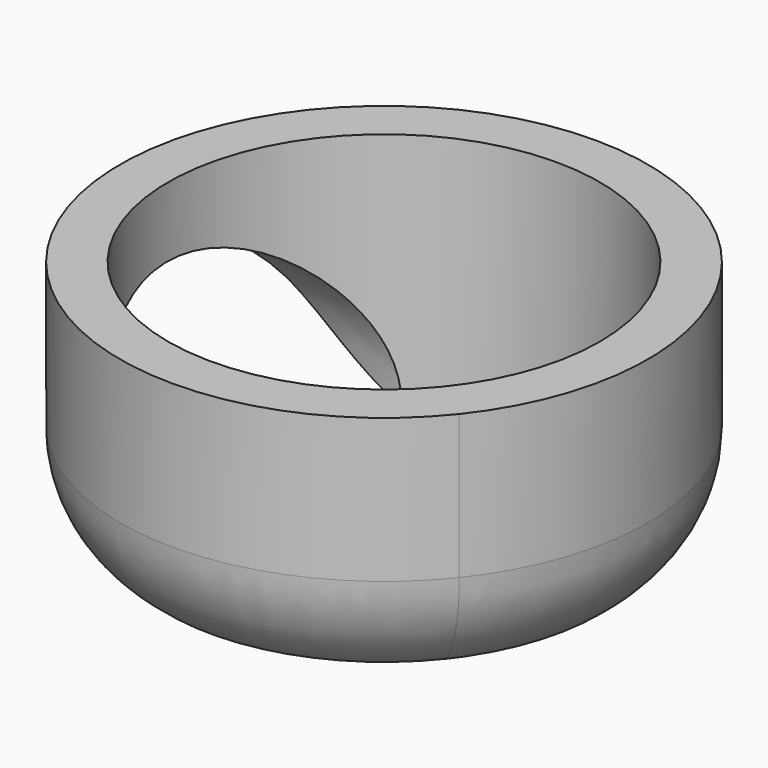
from build123d import *

# Parameters (mm, degrees)
F1_DEPTH    = 10
F3_DEPTH    = 25
F4_DEPTH    = 25
F5_T2_ANGLE = 228.5604314435
F5_T4_ANGLE = 149.7338838055


# Not quite as in the source:
# - a fillet or chamfer that OpenCascade refuses, or shapes differently, is made with other operations: its cross-section is extruded or revolved along the edge and cut away or added


with BuildPart() as f1:
    # F0 (on Top) → F1 (new body)
    with BuildSketch(Plane.XY):
        with BuildLine():
            ThreePointArc((7.4897676428, -4.9903287123), (-9, 0), (7.4897676428, 4.9903287123))
            ThreePointArc((7.4897676428, 4.9903287123), (8.0061615463, 5.944514107), (8.6101788512, 6.8457884973))
            ThreePointArc((8.6101788512, 6.8457884973), (-11, 0), (8.6101788512, -6.8457884973))
            ThreePointArc((8.6101788512, -6.8457884973), (8.0061615463, -5.944514107), (7.4897676428, -4.9903287123))
        make_face()
        with BuildLine():
            ThreePointArc((7.4897676428, 4.9903287123), (8.6141717183, 2.6069226316), (9, 0))
            ThreePointArc((9, 0), (8.6141717183, -2.6069226316), (7.4897676428, -4.9903287123))
            ThreePointArc((7.4897676428, -4.9903287123), (8.0061615463, -5.944514107), (8.6101788512, -6.8457884973))
            ThreePointArc((8.6101788512, -6.8457884973), (11, 0), (8.6101788512, 6.8457884973))
            ThreePointArc((8.6101788512, 6.8457884973), (8.0061615463, 5.944514107), (7.4897676428, 4.9903287123))
        make_face()
    extrude(amount=F1_DEPTH)

    # F2 (on Right) → F3 (cut)
    with BuildSketch(Plane.YZ):
        with BuildLine():
            add(Edge.make_bspline(
                [(-7.6260738851, 0), (-7.6289822236, 4.6128164915), (0.0415342584, 9.6458716707), (7.41270182, 4.5238972991), (7.3739261149, 0)],
                knots=[0, 0, 0, 0, 0.502214143, 1, 1, 1, 1], degree=3))
            Line((-7.6260738851, 0), (7.3739261149, 0))
        make_face()
    extrude(amount=-F3_DEPTH, mode=Mode.SUBTRACT)

    # F2 (on Right) → F4 (cut)
    with BuildSketch(Plane.YZ):
        with BuildLine():
            add(Edge.make_bspline(
                [(-7.6260738851, 0), (-7.6289822236, 4.6128164915), (0.0415342584, 9.6458716707), (7.41270182, 4.5238972991), (7.3739261149, 0)],
                knots=[0, 0, 0, 0, 0.502214143, 1, 1, 1, 1], degree=3))
            Line((-7.6260738851, 0), (7.3739261149, 0))
        make_face()
    extrude(amount=-F4_DEPTH, mode=Mode.SUBTRACT)

    # F5: fillet of radius 5 on 2 edges, made by hand

    # F5_s1 → F5_t2 (revolve, cut)
    with BuildSketch(Plane(origin=(0, 0, 0), x_dir=(0, 0, 1), z_dir=(-0.6223444088, -0.7827435319, 0))):
        with BuildLine():
            ThreePointArc((0, -9), (1.7639320225, -10.472135955), (4, -11))
            Line((4, -11), (0, -11))
            Line((0, -11), (0, -9))
        make_face()
    revolve(axis=Axis((0, 0, 0), (0, 0, 1)), revolution_arc=F5_T2_ANGLE, mode=Mode.SUBTRACT)

    # F5_s3 → F5_t4 (revolve, cut)
    with BuildSketch(Plane(origin=(0, 0, 0), x_dir=(0, 0, 1), z_dir=(0.1429989905, 0.9897228343, 0))):
        with BuildLine():
            ThreePointArc((0, -9), (1.7639320225, -10.472135955), (4, -11))
            Line((4, -11), (0, -11))
            Line((0, -11), (0, -9))
        make_face()
    revolve(axis=Axis((0, 0, 0), (0, 0, 1)), revolution_arc=F5_T4_ANGLE, mode=Mode.SUBTRACT)


solid = f1.part
